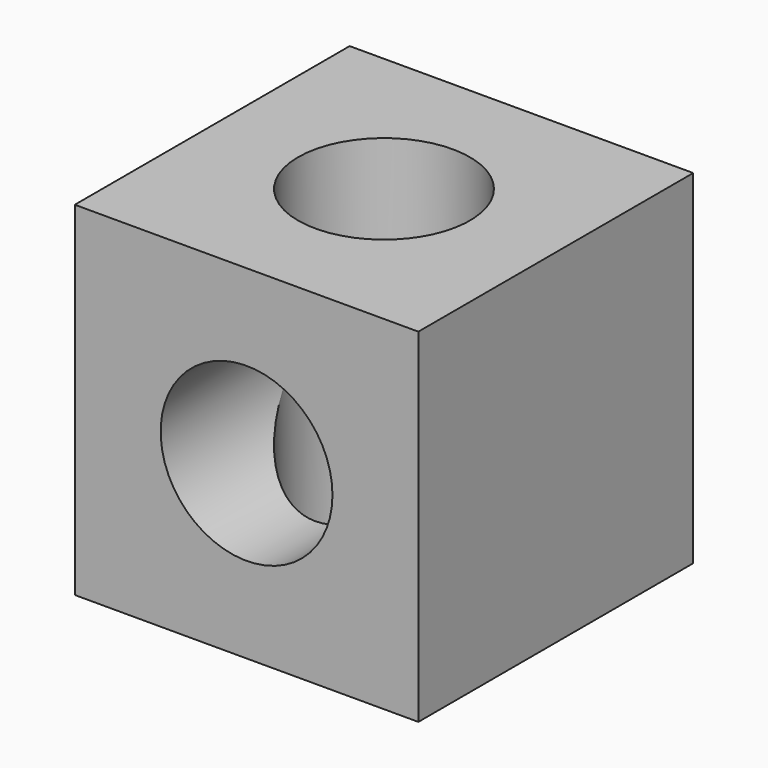
from build123d import *

# Parameters (mm, degrees)
F0_W     = 50.8
F0_H     = 50.8
F0_R     = 12.7
F1_DEPTH = 50.8
F3_D     = 25.4
F5_D     = 25.4


# Not quite as in the source:
# - the program builds the solid bodies; features that only make, move or delete a surface that nothing else refers to are left out


with BuildPart() as f1:
    # F0 (on Right) → F1 (new body)
    with BuildSketch(Plane.YZ):
        Rectangle(F0_W, F0_H)
        Circle(F0_R, mode=Mode.SUBTRACT)
        Circle(F0_R)
    extrude(amount=F1_DEPTH)

    # F3 (through all)
    with Locations(Plane(origin=(0, 25.4, 0), x_dir=(-1, 0, 0), z_dir=(0, 1, 0))):
        with Locations((-25.4, 0)):
            Hole(F3_D / 2)

    # F5 (through all)
    with Locations(Plane.XY.offset(25.4)):
        with Locations((25.4, 0)):
            Hole(F5_D / 2)


solid = f1.part
